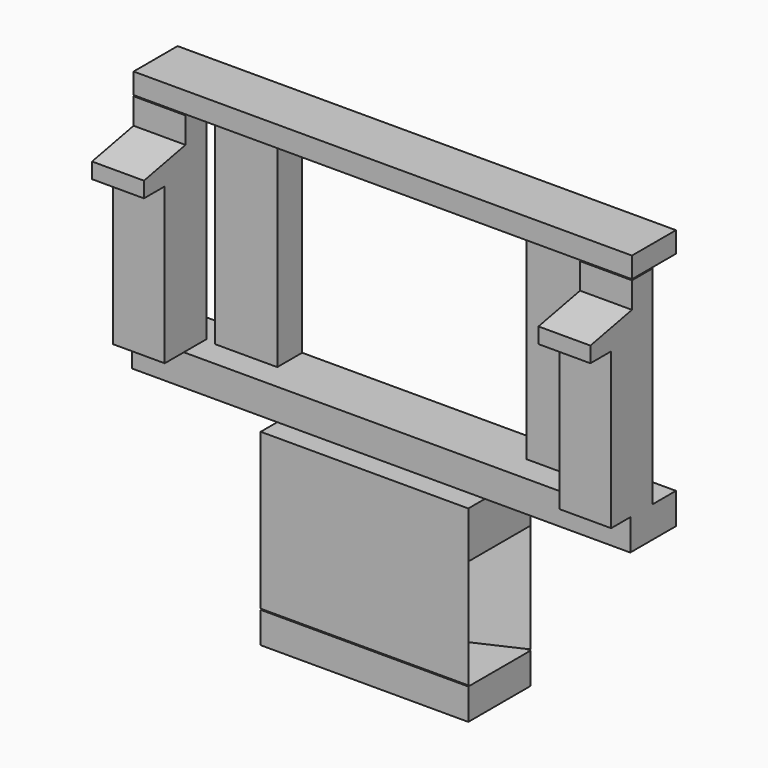
from build123d import *

# Parameters (mm, degrees)
F0_W      = 14
F0_H      = 5.5
F1_DEPTH  = 3
F0_W_2    = 10
F0_H_2    = 2
F2_DEPTH  = 4.5
F4_DEPTH  = 10.5
F5_W      = 6
F5_H      = 3
F5_W_2    = 5
F5_H_2    = 2.7
F5_H_3    = 2.3
F6_DEPTH  = 15
F6_FACE_W = 6
F6_FACE_H = 3
F7_W      = 5
F7_H      = 2.5
F8_DEPTH  = 5
F10_DEPTH = 5
F12_R     = 5
F13_W     = 20
F13_H     = 3
F14_DEPTH = 7.5
F15_W     = 48
F15_H     = 2
F16_DEPTH = 5.3


# Not quite as in the source:
# - a feature names something its author has since deleted; it is built from what else it names


with BuildPart() as f1:
    # F0 (on Top) → F1 (new body)
    with BuildSketch(Plane.XY):
        with Locations((17, 0)):
            Rectangle(F0_W, F0_H)
        Polygon((0, -2.75), (10, -2.75), (10, 2.75), (-10, 2.75), (-10, -2.75), align=None)
    extrude(amount=F1_DEPTH)

    # F0 (on Top) → F2 (join)
    with BuildSketch(Plane.XY):
        Polygon((0, -2.75), (10, -2.75), (10, 2.75), (-10, 2.75), (-10, -2.75), align=None)
        with Locations((-5, -3.75)):
            Rectangle(F0_W_2, F0_H_2)
        with Locations((5, -3.75)):
            Rectangle(F0_W_2, F0_H_2)
    extrude(amount=-F2_DEPTH)

    # F3 (on face) → F4 (join)
    with BuildSketch(Plane(origin=(0, 0, -4.5), x_dir=(1, 0, 0), z_dir=(0, 0, -1))):
        Polygon((0, -2.75), (10, -2.75), (4, 0), (0, 0), align=None)
        Polygon((-10, -2.75), (0, -2.75), (0, 0), (-4, 0), align=None)
        Polygon((4, 2), (10, 4.75), (0, 4.75), (0, 2), align=None)
        Polygon((-4, 2), (0, 2), (0, 4.75), (-10, 4.75), align=None)
    extrude(amount=F4_DEPTH)

    # F5 (on face) → F6 (join)
    with BuildSketch(Plane.XY.offset(3)):
        with Locations((15, 1.25)):
            Rectangle(F5_W, F5_H)
        with Locations((21.5, -1.4)):
            Rectangle(F5_W_2, F5_H_2)
        with Locations((21.5, -3.9)):
            Rectangle(F5_W_2, F5_H_3)
    extrude(amount=F6_DEPTH)

    # F6_face (on face) + F7 (on face) → F8 (join)
    with BuildSketch(Plane(origin=(21.5, -2.55, 18), x_dir=(1, 0, 0), z_dir=(0, 0, 1))):
        with Locations((-6.5, 3.8)):
            Rectangle(F6_FACE_W, F6_FACE_H)
    with BuildSketch(Plane.XY.offset(18)):
        with Locations((21.5, -1.3)):
            Rectangle(F7_W, F7_H)
    extrude(amount=F8_DEPTH)

    # F9 (on face) → F10 (join)
    with BuildSketch(Plane.YZ.offset(24)):
        Polygon((-5.05, 18), (-2.55, 18), (-2.55, 19.5), (-7.55, 19.5), (-7.55, 18), align=None)
        Polygon((-7.55, 19.5), (-2.55, 19.5), (-2.55, 20.5), align=None)
    extrude(amount=-F10_DEPTH)

    # F11: F1 across plane


with BuildPart() as f1_1:
    add(f1.part)
    add(f1.part.mirror(Plane.YZ))

    # F12
    f12_edges = [f1_1.edges().sort_by_distance(p)[0] for p in [
        (-4, -2, -9.75),
        (4, -2, -9.75),
        (4, 0, -9.75),
        (-4, 0, -9.75),
    ]]
    fillet(f12_edges, radius=F12_R)


with BuildPart() as f14:
    # F13 (on face) → F14 (new body)
    with BuildSketch(Plane.XZ.offset(4.75)):
        with Locations((0, -16.6)):
            Rectangle(F13_W, F13_H)
    extrude(amount=-F14_DEPTH)


with BuildPart() as f16:
    # F15 (on face) → F16 (new body)
    with BuildSketch(Plane.XZ.offset(2.55)):
        with Locations((0, 24.1)):
            Rectangle(F15_W, F15_H)
    extrude(amount=-F16_DEPTH)


solid = Compound([f1_1.part, f14.part, f16.part])
